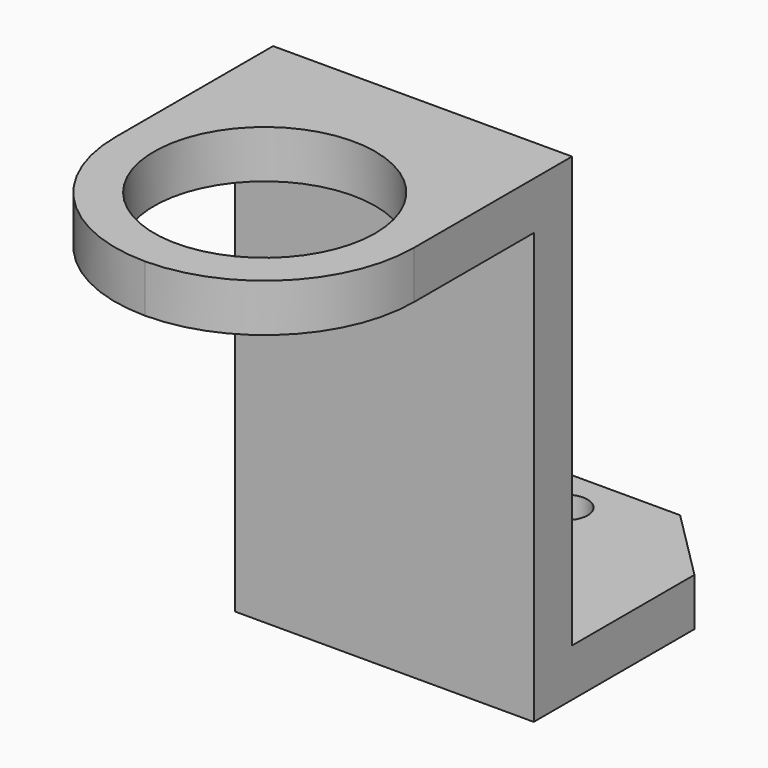
from build123d import *

# Parameters (mm, degrees)
F0_W     = 25
F0_H     = 18.8
F0_R     = 1.8
F1_DEPTH = 4
F0_H_2   = 4
F2_DEPTH = 40
F3_W     = 25
F3_H     = 4
F4_DEPTH = 25
F5_R     = 9.25
F6_DEPTH = 4
F7_R     = 12.49999
F8_SIZE  = 6


# Not quite as in the source:
# - a fillet or chamfer is up to 0.001 mm smaller than in the source, because OpenCascade refuses the exact size


with BuildPart() as f1:
    # F0 (on Top) → F1 (new body)
    with BuildSketch(Plane.XY):
        with Locations((0, -9.4)):
            Rectangle(F0_W, F0_H)
        with Locations((0, -3.8)):
            Circle(F0_R, mode=Mode.SUBTRACT)
    extrude(amount=F1_DEPTH)

    # F0 (on Top) → F2 (join)
    with BuildSketch(Plane.XY):
        with Locations((0, -20.8)):
            Rectangle(F0_W, F0_H_2)
    extrude(amount=F2_DEPTH)

    # F3 (on face) → F4 (join)
    with BuildSketch(Plane.XZ.offset(22.8)):
        with Locations((0, 38)):
            Rectangle(F3_W, F3_H)
    extrude(amount=F4_DEPTH)

    # F5 (on face) → F6 (cut, through all)
    with BuildSketch(Plane(origin=(0, 0, 36), x_dir=(1, 0, 0), z_dir=(0, 0, -1))):
        with Locations((0, 35.3)):
            Circle(F5_R)
    extrude(amount=-F6_DEPTH, mode=Mode.SUBTRACT)

    # F7 (radius 12.5 in the source; OpenCascade refuses exactly that, so slightly less here)
    f7_edges = [f1.edges().sort_by_distance(p)[0] for p in [
        (12.5, -47.8, 38),
        (-12.5, -47.8, 38),
    ]]
    fillet(f7_edges, radius=F7_R)

    # F8
    f8_edges = [f1.edges().sort_by_distance(p)[0] for p in [
        (12.5, 0, 2),
        (-12.5, 0, 2),
    ]]
    chamfer(f8_edges, length=F8_SIZE)


solid = f1.part
